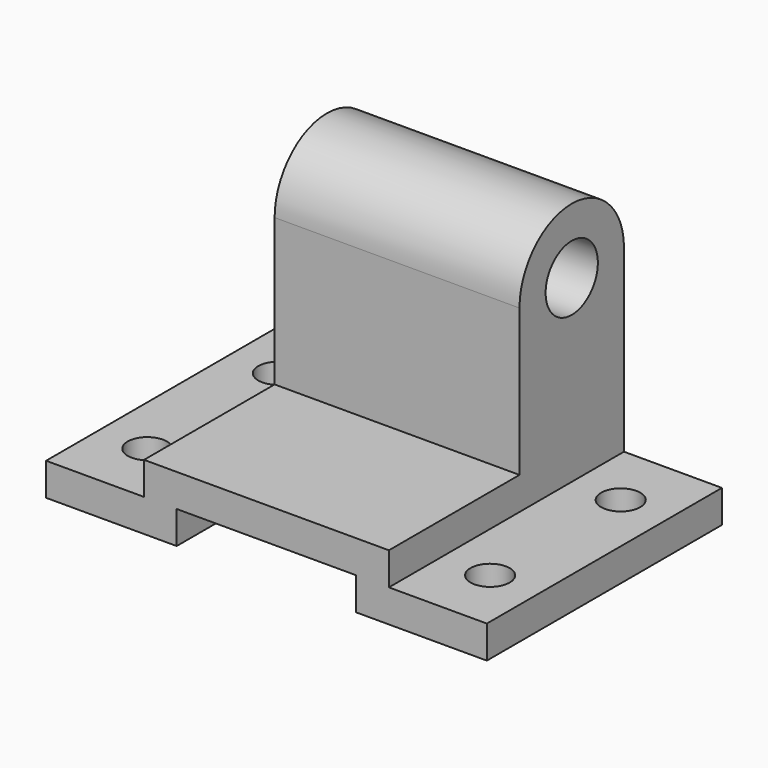
from build123d import *

# Parameters (mm, degrees)
F1_DEPTH = 228.6
F2_W     = 190.5
F2_H     = 101.6
F3_DEPTH = 114.3
F5_DEPTH = 190.5
F8_D     = 50.8
F10_D    = 30.48


with BuildPart() as f1:
    # F0 (on Front) → F1 (new body)
    with BuildSketch(Plane.XZ):
        Polygon((-69.85, 25.4), (0, 25.4), (69.85, 25.4), (69.85, 0), (171.45, 0), (171.45, 25.4), (95.25, 25.4), (95.25, 50.8), (0, 50.8), (-95.25, 50.8), (-95.25, 25.4), (-171.45, 25.4), (-171.45, 0), (-69.85, 0), align=None)
    extrude(amount=F1_DEPTH)

    # F2 (on face) → F3 (join)
    with BuildSketch(Plane.XY.offset(50.8)):
        with Locations((0, -50.8)):
            Rectangle(F2_W, F2_H)
    extrude(amount=F3_DEPTH)

    # F4 (on face) → F5 (join)
    with BuildSketch(Plane.YZ.offset(95.25)):
        with BuildLine():
            Line((-101.6, 165.1), (0, 165.1))
            ThreePointArc((0, 165.1), (-50.8, 215.9), (-101.6, 165.1))
        make_face()
        with BuildLine():
            Line((0, 25.4), (0, 165.1))
            ThreePointArc((0, 165.1), (-50.8, 114.3), (-101.6, 165.1))
            Line((-101.6, 165.1), (-101.6, 50.8))
            Line((-101.6, 50.8), (-228.6, 50.8))
            Line((-228.6, 50.8), (-228.6, 25.4))
            Line((-228.6, 25.4), (0, 25.4))
        make_face()
    extrude(amount=-F5_DEPTH)

    # F8 (through all)
    with Locations(Plane.YZ.offset(95.25)):
        with Locations((-50.8, 165.1)):
            Hole(F8_D / 2)

    # F10 (through all)
    with Locations(Plane.XY.offset(25.4)):
        with Locations((-133.35, -50.8), (133.35, -50.8), (-133.35, -177.8), (133.35, -177.8)):
            Hole(F10_D / 2)


solid = f1.part
